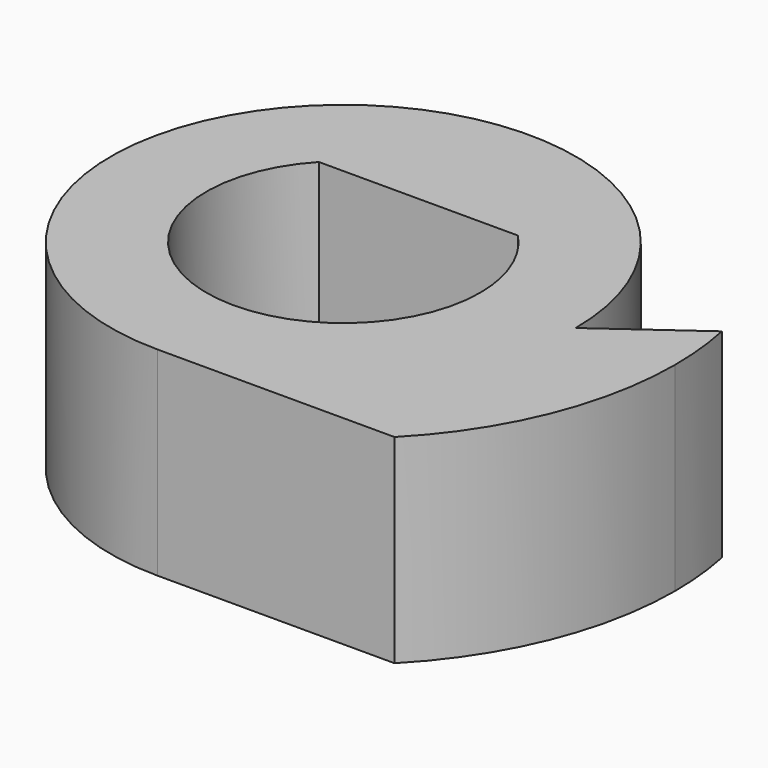
from build123d import *

# Parameters (mm, degrees)
F1_DEPTH = 6


# Not quite as in the source:
# - a feature names something its author has since deleted; it is built from what else it names


with BuildPart() as f1:
    # F0 (on Top) → F1 (new body)
    with BuildSketch(Plane.XY):
        with BuildLine():
            ThreePointArc((0, -7), (4.9497474683, -4.9497474683), (7, 0))
            ThreePointArc((7, 0), (-4.9497474683, 4.9497474683), (0, -7))
        make_face()
        with BuildLine():
            ThreePointArc((3, 2.8311879132), (3.8334465563, 1.5232572009), (4.125, 0))
            ThreePointArc((4.125, 0), (-1.5232572009, -3.8334465563), (-3, 2.8311879132))
            ThreePointArc((-3, 2.8311879132), (0, 4.125), (3, 2.8311879132))
        make_face(mode=Mode.SUBTRACT)
        with BuildLine():
            Line((-3, 2.8311879132), (3, 2.8311879132))
            ThreePointArc((3, 2.8311879132), (0, 4.125), (-3, 2.8311879132))
        make_face()
        with BuildLine():
            ThreePointArc((7.1414284285, -7), (9.2578151927, -3.7805896177), (10, 0))
            ThreePointArc((10, 0), (9.9484557051, 1.0140163134), (9.7943541832, 2.0175792755))
            Line((9.7943541832, 2.0175792755), (7, 0))
            ThreePointArc((7, 0), (4.9497474683, -4.9497474683), (0, -7))
            Line((0, -7), (7.1414284285, -7))
        make_face()
    extrude(amount=F1_DEPTH)


solid = f1.part
